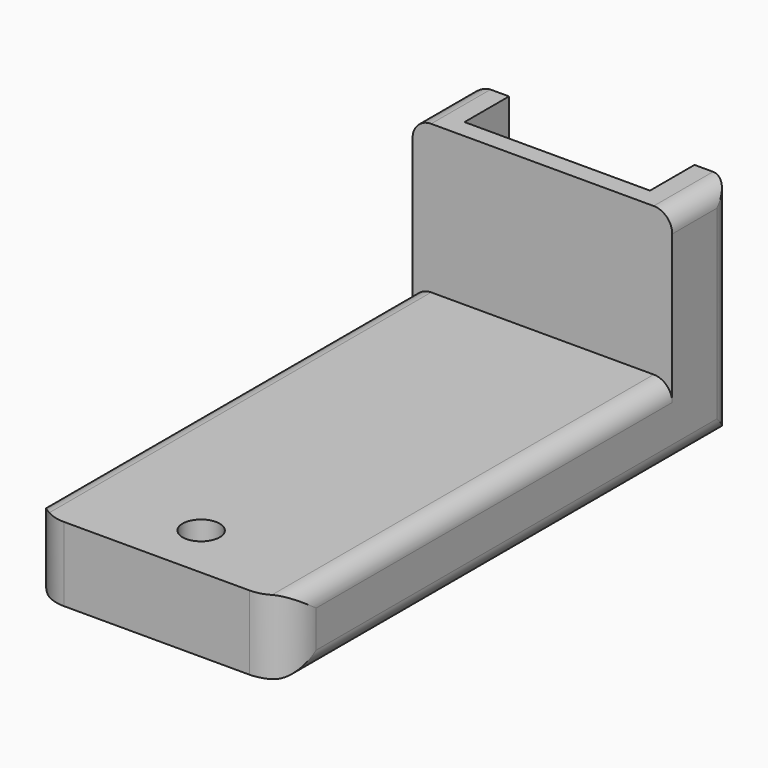
from build123d import *

# Parameters (mm, degrees)
F0_W        = 14
F0_H        = 30
F0_R        = 1
F1_DEPTH    = 4
F3_DEPTH    = 8
F4_DEPTH    = 4.001
F5_R        = 1
F6_T1_DEPTH = 12


# Not quite as in the source:
# - a fillet or chamfer that OpenCascade refuses, or shapes differently, is made with other operations: its cross-section is extruded or revolved along the edge and cut away or added


with BuildPart() as f1:
    # F0 (on Top) → F1 (new body)
    with BuildSketch(Plane.XY):
        with Locations((0, 15)):
            Rectangle(F0_W, F0_H)
        with Locations((0, 3)):
            Circle(F0_R, mode=Mode.SUBTRACT)
    extrude(amount=F1_DEPTH)

    # F2 (on face) → F3 (join)
    with BuildSketch(Plane.XY.offset(4)):
        Polygon((-5, 27), (-5, 30), (-7, 30), (-7, 26), (7, 26), (7, 30), (5, 30), (5, 27), align=None)
    extrude(amount=F3_DEPTH)

    # F4 (cut, through all): a face of the model
    f4_faces = [f1.faces().sort_by_distance(p)[0] for p in [
        (0, 28.5, 4),
    ]]
    extrude(f4_faces, amount=-F4_DEPTH, mode=Mode.SUBTRACT)

    # F5
    f5_edges = [f1.edges().sort_by_distance(p)[0] for p in [
        (-7, 30, 6),
        (7, 30, 6),
        (-7, 28, 12),
        (7, 28, 12),
        (7, 15, 0),
        (-7, 15, 0),
        (-7, 13, 4),
        (7, 13, 4),
    ]]
    fillet(f5_edges, radius=F5_R)

    # F6: fillet of radius 2 on 2 edges, made by hand

    # F6_s2 → F6_t1 (cut)
    with BuildSketch(Plane.XY.offset(-4)):
        with BuildLine():
            ThreePointArc((-7, 2), (-6.4142135624, 0.5857864376), (-5, 0))
            Line((-5, 0), (-7, 0))
            Line((-7, 0), (-7, 2))
        make_face()
        with BuildLine():
            ThreePointArc((5, 0), (6.4142135624, 0.5857864376), (7, 2))
            Line((7, 2), (7, 0))
            Line((7, 0), (5, 0))
        make_face()
    extrude(amount=F6_T1_DEPTH, mode=Mode.SUBTRACT)


solid = f1.part
